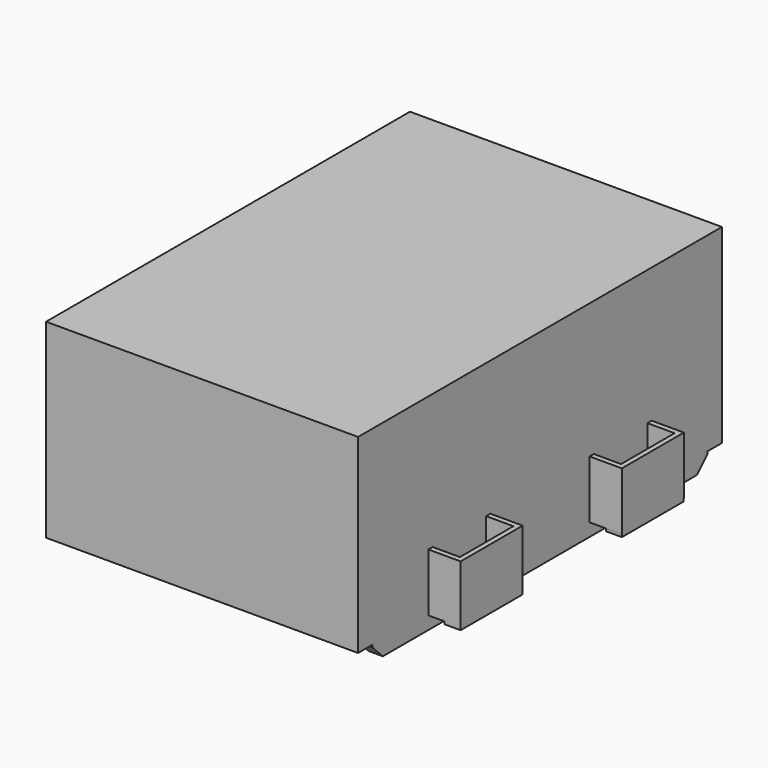
from build123d import *

# Parameters (mm, degrees)
F0_W          = 60.96
F0_H          = 91.44
F0_W_2        = 50.8
F0_H_2        = 86.614
F1_DEPTH      = 28.448
F3_DEPTH      = 25.4
F4_W          = 66.649839282
F4_H          = 6.9823637605
F5_DEPTH      = 3.048
F6_W          = 64.9686481762
F6_H          = 4.777956934
F7_DEPTH      = 3.048
F9_DEPTH      = 2.286
F10_W         = 99.848318845
F10_H         = 48.2080141082
F11_DEPTH     = 50.8
F13_T1_DEPTH  = 15.8581495789
F13_T3_DEPTH  = 15.8581495789
F13_T8_DEPTH  = 41.5121495789
F13_T13_DEPTH = 41.5121495789
F13_T18_DEPTH = 41.5121495789
F13_T23_DEPTH = 41.5121495789
F14_W         = 15.24
F14_H         = 23.368
F15_DEPTH     = 6.35
F16_W         = 5.3607832682
F16_H         = 13.1506472826
F17_DEPTH     = 25.909
F19_DEPTH     = 0.254
F20_DEPTH     = 0.254
F21_DEPTH     = 1.016
F22_W         = 3.175
F22_H         = 15.24
F22_H_2       = 15.425526537
F23_DEPTH     = 0.508
F24_W         = 3.175
F24_H         = 15.24
F24_H_2       = 15.1729788631
F25_DEPTH     = 0.508
F26_W         = 1.4869117904
F26_H         = 15.24
F26_H_2       = 15.1544166729
F27_DEPTH     = 0.508
F28_W         = 1.5113
F28_H         = 15.24
F28_W_2       = 1.492887156
F28_H_2       = 15.3870563954
F29_DEPTH     = 0.254
F30_DEPTH     = 0.381
F31_DEPTH     = 0.254
F32_W         = 105.9566885233
F32_H         = 116.2753328681
F33_DEPTH     = 14.5
F35_DEPTH     = 25
F36_DEPTH     = 1
F37_DEPTH     = 0.4
F38_DEPTH     = 0.4
F39_W         = 61.341
F39_H         = 89.424
F40_DEPTH     = 1.5
F41_T4_DEPTH  = 72.4640866379
F41_T9_DEPTH  = 72.4640866379


# Not quite as in the source:
# - a fillet or chamfer that OpenCascade refuses, or shapes differently, is made with other operations: its cross-section is extruded or revolved along the edge and cut away or added
# - a feature names something its author has since deleted; it is built from what else it names


with BuildPart() as f1:
    # F0 (on Top) → F1 (new body)
    with BuildSketch(Plane.XY):
        Rectangle(F0_W, F0_H)
        Rectangle(F0_W_2, F0_H_2, mode=Mode.SUBTRACT)
    extrude(amount=F1_DEPTH)

    # F2 (on face) → F3 (cut)
    with BuildSketch(Plane(origin=(0, 45.72, 0), x_dir=(-1, 0, 0), z_dir=(0, 1, 0))):
        Polygon((-9.4803553075, 0), (0, 0), (9.4803553075, 0), (5.461, 8.763), (-5.461, 8.763), align=None)
        Polygon((-9.4803553075, 28.448), (-5.461, 19.685), (5.461, 19.685), (9.4803553075, 28.448), (0, 28.448), align=None)
    extrude(amount=-F3_DEPTH, mode=Mode.SUBTRACT)

    # F4 (on Top) → F5 (cut)
    with BuildSketch(Plane.XY):
        with Locations((-0.1057945192, 44.6448102593)):
            Rectangle(F4_W, F4_H)
        with Locations((-0.1057945192, -44.6448102593)):
            Rectangle(F4_W, F4_H)
    extrude(amount=F5_DEPTH, mode=Mode.SUBTRACT)

    # F6 (on face) → F7 (cut)
    with BuildSketch(Plane.XY.offset(28.448)):
        with Locations((-2.0043240881, 43.331021533)):
            Rectangle(F6_W, F6_H)
        with Locations((-2.0043240881, -43.331021533)):
            Rectangle(F6_W, F6_H)
    extrude(amount=-F7_DEPTH, mode=Mode.SUBTRACT)

    # F8 (on face) → F9 (cut)
    with BuildSketch(Plane(origin=(25.4, 0, 0), x_dir=(0, -1, 0), z_dir=(-1, 0, 0))):
        Polygon((-43.0863499641, 0), (-41.1536283791, 0), (-25.9136283791, 0), (-25.9136283791, 30.48), (-41.1536283791, 30.48), (-43.0863499641, 30.48), align=None)
        Polygon((25.9136283791, 30.48), (25.9136283791, 0), (41.1536283791, 0), (43.0863499641, 0), (43.0863499641, 30.48), (41.1536283791, 30.48), align=None)
    extrude(amount=-F9_DEPTH, mode=Mode.SUBTRACT)

    # F10 (on Right) → F11 (cut)
    with BuildSketch(Plane.YZ):
        with Locations((1.7518345267, 13.4315635078)):
            Rectangle(F10_W, F10_H)
    extrude(amount=-F11_DEPTH, mode=Mode.SUBTRACT)

    # F12: F1 across plane


with BuildPart() as f1_1:
    add(f1.part)
    add(f1.part.mirror(Plane.YZ))

    # F13: chamfer of 2.54 on 12 edges, made by hand

    # F13_s2 → F13_t1 (cut)
    with BuildSketch(Plane.YZ.offset(-37.0120747894)):
        Polygon((38.402043066, 28.448), (40.942043066, 25.908), (40.942043066, 28.448), align=None)
        Polygon((38.6136283791, 0), (41.1536283791, 2.54), (41.1536283791, 0), align=None)
        Polygon((-40.942043066, 25.908), (-38.402043066, 28.448), (-40.942043066, 28.448), align=None)
        Polygon((-38.6136283791, 0), (-41.1536283791, 2.54), (-41.1536283791, 0), align=None)
    extrude(amount=F13_T1_DEPTH, mode=Mode.SUBTRACT)

    # F13_s4 → F13_t3 (cut)
    with BuildSketch(Plane.YZ.offset(21.1539252106)):
        Polygon((38.402043066, 28.448), (40.942043066, 25.908), (40.942043066, 28.448), align=None)
        Polygon((-40.942043066, 25.908), (-38.402043066, 28.448), (-40.942043066, 28.448), align=None)
        Polygon((-38.6136283791, 0), (-41.1536283791, 2.54), (-41.1536283791, 0), align=None)
        Polygon((38.6136283791, 0), (41.1536283791, 2.54), (41.1536283791, 0), align=None)
    extrude(amount=F13_T3_DEPTH, mode=Mode.SUBTRACT)


with BuildPart() as f13_tool6:
    # F13_s7 → F13_t8 (new body)
    with BuildSketch(Plane.XY.offset(-6.5320747894)):
        Polygon((25.4, 23.3736283791), (27.94, 25.9136283791), (25.4, 25.9136283791), align=None)
    extrude(amount=F13_T8_DEPTH)

    split(bisect_by=Plane.YZ.offset(27.686), keep=Keep.BOTTOM)


with BuildPart() as f1_2:
    add(f1_1.part)

    # F13_t5: cut F13_tool6
    add(f13_tool6.part, mode=Mode.SUBTRACT)


with BuildPart() as f13_tool11:
    # F13_s12 → F13_t13 (new body)
    with BuildSketch(Plane.XY.offset(34.9800747894)):
        Polygon((25.4, -23.3736283791), (27.94, -25.9136283791), (25.4, -25.9136283791), align=None)
    extrude(amount=-F13_T13_DEPTH)

    split(bisect_by=Plane.YZ.offset(27.686), keep=Keep.BOTTOM)


with BuildPart() as f1_3:
    add(f1_2.part)

    # F13_t10: cut F13_tool11
    add(f13_tool11.part, mode=Mode.SUBTRACT)


with BuildPart() as f13_tool16:
    # F13_s17 → F13_t18 (new body)
    with BuildSketch(Plane.XY.offset(-6.5320747894)):
        Polygon((-27.94, 25.9136283791), (-25.4, 23.3736283791), (-25.4, 25.9136283791), align=None)
    extrude(amount=F13_T18_DEPTH)

    split(bisect_by=Plane.YZ.offset(-27.686), keep=Keep.TOP)


with BuildPart() as f1_4:
    add(f1_3.part)

    # F13_t15: cut F13_tool16
    add(f13_tool16.part, mode=Mode.SUBTRACT)


with BuildPart() as f13_tool21:
    # F13_s22 → F13_t23 (new body)
    with BuildSketch(Plane.XY.offset(34.9800747894)):
        Polygon((-25.4, -23.3736283791), (-27.94, -25.9136283791), (-25.4, -25.9136283791), align=None)
    extrude(amount=-F13_T23_DEPTH)

    split(bisect_by=Plane.YZ.offset(-27.686), keep=Keep.TOP)


with BuildPart() as f1_5:
    add(f1_4.part)

    # F13_t20: cut F13_tool21
    add(f13_tool21.part, mode=Mode.SUBTRACT)

    # F14 (on face) → F15 (join)
    with BuildSketch(Plane.YZ.offset(30.48)):
        with Locations((-19.812, 14.224)):
            Rectangle(F14_W, F14_H)
        with Locations((19.812, 14.224)):
            Rectangle(F14_W, F14_H)
    extrude(amount=F15_DEPTH)

    # F16 (on face) → F17 (cut, through all)
    with BuildSketch(Plane.XY.offset(25.908)):
        with Locations((33.1603916341, -19.8066011071)):
            Rectangle(F16_W, F16_H)
        with Locations((33.1603916341, 19.8066011071)):
            Rectangle(F16_W, F16_H)
    extrude(amount=-F17_DEPTH, mode=Mode.SUBTRACT)

    # F18: F1 across plane


with BuildPart() as f1_6:
    add(f1_5.part)
    add(f1_5.part.mirror(Plane.YZ))

    # F19 (cut): faces of the model
    f19_faces = [f1_6.faces().sort_by_distance(p)[0] for p in [
        (26.543, -43.0863499641, 14.224),
        (-26.543, -43.0863499641, 14.224),
    ]]
    extrude(f19_faces, amount=-F19_DEPTH, mode=Mode.SUBTRACT)

    # F20 (cut): faces of the model
    f20_faces = [f1_6.faces().sort_by_distance(p)[0] for p in [
        (26.543, 43.0863499641, 14.224),
        (-26.543, 43.0863499641, 14.224),
    ]]
    extrude(f20_faces, amount=-F20_DEPTH, mode=Mode.SUBTRACT)

    # F21 (cut): a face of the model
    f21_faces = [f1_6.faces().sort_by_distance(p)[0] for p in [
        (0, -45.72, 14.224),
    ]]
    extrude(f21_faces, amount=-F21_DEPTH, mode=Mode.SUBTRACT)

    # F22 (on face) → F23 (join)
    with BuildSketch(Plane.XY.offset(25.908)):
        with Locations((-35.2425, 19.812)):
            Rectangle(F22_W, F22_H)
        with Locations((-35.2425, -19.7230628692)):
            Rectangle(F22_W, F22_H_2)
    extrude(amount=F23_DEPTH)

    # F24 (on face) → F25 (join)
    with BuildSketch(Plane(origin=(0, 0, 2.54), x_dir=(1, 0, 0), z_dir=(0, 0, -1))):
        with Locations((35.2425, 19.812)):
            Rectangle(F24_W, F24_H)
        with Locations((35.2425, -19.7903430089)):
            Rectangle(F24_W, F24_H_2)
    extrude(amount=F25_DEPTH)

    # F26 (on face) → F27 (join)
    with BuildSketch(Plane.XY.offset(25.908)):
        with Locations((36.0865441048, -19.812)):
            Rectangle(F26_W, F26_H)
        with Locations((36.0865441048, 19.7994005866)):
            Rectangle(F26_W, F26_H_2)
    extrude(amount=F27_DEPTH)

    # F28 (on face) → F29 (join)
    with BuildSketch(Plane(origin=(0, 0, 2.54), x_dir=(1, 0, 0), z_dir=(0, 0, -1))):
        with Locations((-36.07435, 19.812)):
            Rectangle(F28_W, F28_H)
        with Locations((-36.083556422, -19.7531366721)):
            Rectangle(F28_W_2, F28_H_2)
    extrude(amount=F29_DEPTH)

    # F30 (add): faces of the model
    f30_faces = [f1_6.faces().sort_by_distance(p)[0] for p in [
        (-30.48, 0.4258489378, 14.2172059936),
        (-35.3187, -19.812, 2.413),
        (-35.8407832682, -19.8066011071, 14.224),
        (-36.83, -19.8101053315, 14.3540262363),
    ]]
    extrude(f30_faces, amount=F30_DEPTH, dir=(-1, 0, 0))

    # F31 (add): a face of the model
    f31_faces = [f1_6.faces().sort_by_distance(p)[0] for p in [
        (-35.337112844, 19.7531366721, 2.413),
    ]]
    extrude(f31_faces, amount=F31_DEPTH)

    # F32 (on face) → F33 (cut)
    with BuildSketch(Plane.XY.offset(28.448)):
        with Locations((11.0789313912, -7.9427920282)):
            Rectangle(F32_W, F32_H)
    extrude(amount=-F33_DEPTH, mode=Mode.SUBTRACT)

    # F34 (on face) → F35 (join)
    with BuildSketch(Plane.XY.offset(13.948)):
        Polygon((-30.861, -27.432), (-30.861, -44.704), (30.48, -44.704), (30.48, -27.432), (30.48, -26.3819247484), (30.48, -13.2312774658), (30.48, -12.192), (30.48, 12.192), (30.48, 13.2312774658), (30.48, 26.3819247484), (30.48, 27.432), (30.48, 45.72), (-30.861, 45.72), (-30.861, 27.432), (-30.861, 26.3819247484), (-30.861, 13.2312774658), (-30.861, 12.192), (-30.861, -12.192), (-30.861, -13.2312774658), (-30.861, -26.3819247484), align=None)
        Polygon((-25.4, -43.3403499641), (-27.686, -43.3403499641), (-27.686, -25.6596283791), (-27.686, 25.6596283791), (-27.686, 43.3403499641), (-25.4, 43.3403499641), (25.4, 43.3403499641), (27.686, 43.3403499641), (27.686, 25.6596283791), (27.686, -25.6596283791), (27.686, -43.3403499641), (25.4, -43.3403499641), align=None, mode=Mode.SUBTRACT)
    extrude(amount=F35_DEPTH)

    # F36 (cut): a face of the model
    f36_faces = [f1_6.faces().sort_by_distance(p)[0] for p in [
        (-0.1974395314, 45.72, 21.5545051375),
    ]]
    extrude(f36_faces, amount=-F36_DEPTH, mode=Mode.SUBTRACT)

    # F37 (add): a face of the model
    f37_faces = [f1_6.faces().sort_by_distance(p)[0] for p in [
        (-35.083112844, 19.7531366721, 2.413),
    ]]
    extrude(f37_faces, amount=F37_DEPTH)

    # F38 (add): a face of the model
    f38_faces = [f1_6.faces().sort_by_distance(p)[0] for p in [
        (-35.3187, -19.812, 2.413),
    ]]
    extrude(f38_faces, amount=F38_DEPTH)

    # F39 (on face) → F40 (join)
    with BuildSketch(Plane.XY.offset(38.948)):
        with Locations((-0.1905, 0.008)):
            Rectangle(F39_W, F39_H)
    extrude(amount=F40_DEPTH)

    # F41: chamfer of 5 on 2 edges, made by hand


with BuildPart() as f41_tool2:
    # F41_s3 → F41_t4 (new body)
    with BuildSketch(Plane.XZ.offset(-36.2320433189)):
        Polygon((25.4, 8.948), (30.4, 13.948), (25.4, 13.948), align=None)
    extrude(amount=F41_T4_DEPTH)

    split(bisect_by=Plane.YZ.offset(27.686), keep=Keep.BOTTOM)


with BuildPart() as f1_7:
    add(f1_6.part)

    # F41_t1: cut F41_tool2
    add(f41_tool2.part, mode=Mode.SUBTRACT)


with BuildPart() as f41_tool7:
    # F41_s8 → F41_t9 (new body)
    with BuildSketch(Plane.XZ.offset(-36.2320433189)):
        Polygon((-25.4, 8.948), (-30.4, 13.948), (-25.4, 13.948), align=None)
    extrude(amount=F41_T9_DEPTH)

    split(bisect_by=Plane.YZ.offset(-27.686), keep=Keep.TOP)


with BuildPart() as f1_8:
    add(f1_7.part)

    # F41_t6: cut F41_tool7
    add(f41_tool7.part, mode=Mode.SUBTRACT)


solid = f1_8.part
